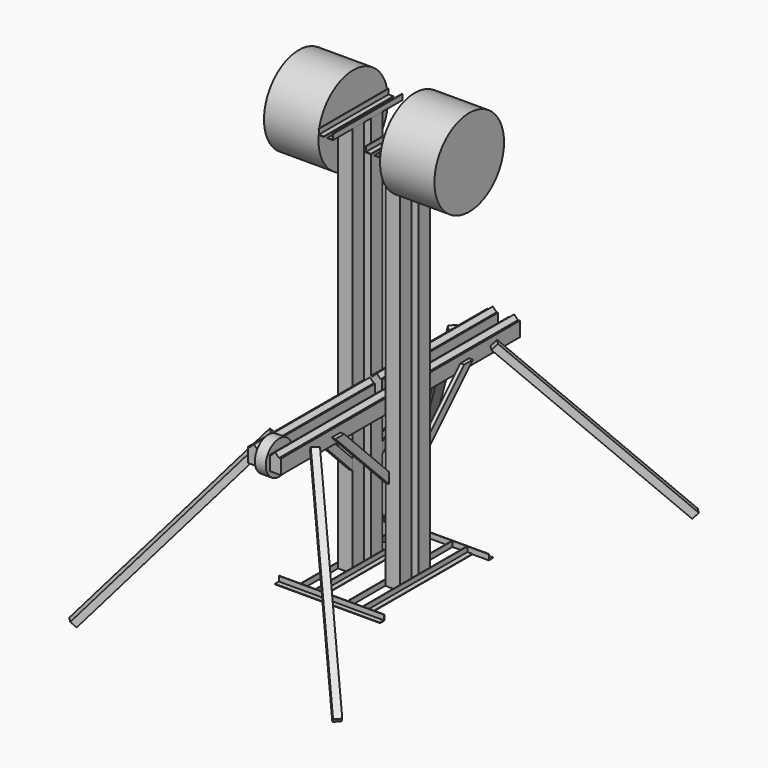
from build123d import *

# Parameters (mm, degrees)
F0_W      = 101.6
F0_H      = 101.6
F1_DEPTH  = 2743.2
F3_DEPTH  = 1016
F6_DEPTH  = 76.2
F8_DEPTH  = 26.924
F12_DEPTH = 457.2
F14_DEPTH = 368.3
F17_DEPTH = 304.8
F15_R     = 30.1625
F18_DEPTH = 381
F22_DEPTH = 50.8


with BuildPart() as f1:
    # F0 (on Top) → F1 (new body)
    with BuildSketch(Plane.XY):
        with Locations((-165.1, -80.9625)):
            Rectangle(F0_W, F0_H)
    extrude(amount=F1_DEPTH)


with BuildPart() as f1b:
    # F0 (on Top) → F1, piece 2 (new body)
    with BuildSketch(Plane.XY):
        with Locations((-165.1, 80.9625)):
            Rectangle(F0_W, F0_H)
    extrude(amount=F1_DEPTH)


with BuildPart() as f1c:
    # F0 (on Top) → F1, piece 3 (new body)
    with BuildSketch(Plane.XY):
        with Locations((165.1, 80.9625)):
            Rectangle(F0_W, F0_H)
    extrude(amount=F1_DEPTH)


with BuildPart() as f1d:
    # F0 (on Top) → F1, piece 4 (new body)
    with BuildSketch(Plane.XY):
        with Locations((165.1, -80.9625)):
            Rectangle(F0_W, F0_H)
    extrude(amount=F1_DEPTH)


with BuildPart() as f3:
    # F2 (on face) → F3 (new body)
    with BuildSketch(Plane.XZ.offset(-30.1625)):
        Polygon((-101.6, 1155.7), (-114.3, 1155.7), (-114.3, 1054.1), (-38.1, 1054.1), (-38.1, 1155.7), (-47.7184632736, 1155.7), align=None)
        Polygon((-74.6592316368, 1182.6407683632), (-101.6, 1155.7), (-47.7184632736, 1155.7), align=None)
    extrude(amount=-F3_DEPTH)


with BuildPart() as f3b:
    # F2 (on face) → F3, piece 2 (new body)
    with BuildSketch(Plane.XZ.offset(-30.1625)):
        Polygon((114.3, 1054.1), (114.3, 1155.7), (101.6, 1155.7), (47.7184632736, 1155.7), (38.1, 1155.7), (38.1, 1054.1), align=None)
        Polygon((47.7184632736, 1155.7), (101.6, 1155.7), (74.6592316368, 1182.6407683632), align=None)
    extrude(amount=-F3_DEPTH)


with BuildPart() as f4_1:
    # F4: instance of F3b
    add(f3b.part.mirror(Plane.XZ))


with BuildPart() as f4_2:
    # F4: instance of F3
    add(f3.part.mirror(Plane.XZ))


with BuildPart() as f6:
    # F5 (on face) → F6 (new body)
    with BuildSketch(Plane.YZ.offset(-38.1)):
        with BuildLine():
            ThreePointArc((-859.2767465332, 1054.1), (-850.6493347335, 1078.8515698747), (-847.725, 1104.9))
            ThreePointArc((-847.725, 1104.9), (-850.6493347335, 1130.9484301253), (-859.2767465332, 1155.7))
            Line((-859.2767465332, 1155.7), (-1046.1625, 1155.7))
            Line((-1046.1625, 1155.7), (-1046.1625, 1054.1))
            Line((-1046.1625, 1054.1), (-859.2767465332, 1054.1))
        make_face()
        with BuildLine():
            Line((-1046.1625, 1155.7), (-859.2767465332, 1155.7))
            ThreePointArc((-859.2767465332, 1155.7), (-1082.675, 1104.9), (-859.2767465332, 1054.1))
            Line((-859.2767465332, 1054.1), (-1046.1625, 1054.1))
            Line((-1046.1625, 1054.1), (-1046.1625, 1155.7))
        make_face()
    extrude(amount=F6_DEPTH)


with BuildPart() as f8:
    # F7 (on face) → F8 (new body)
    with BuildSketch(Plane.YZ.offset(114.3)):
        Polygon((-550.8625, 1054.1), (-131.7625, 635), (-131.7625, 711.1884929312), (-474.6740070688, 1054.1), align=None)
        Polygon((-601.6625, 1104.9), (-550.8625, 1054.1), (-474.6740070688, 1054.1), (-525.4740070688, 1104.9), align=None)
    extrude(amount=F8_DEPTH)


with BuildPart() as f9_1:
    # F9: instance of F8
    add(f8.part.mirror(Plane.XZ))


with BuildPart() as f10_1:
    # F10: instance of F8
    add(f8.part.mirror(Plane.YZ))


with BuildPart() as f10_2:
    # F10: instance of F9_1
    add(f9_1.part.mirror(Plane.YZ))


with BuildPart() as f12:
    # F11 (on Front) → F12 (new body, symmetric)
    with BuildSketch(Plane.XZ):
        Polygon((-254, 0), (-215.9, 0), (-215.9, 38.1), (-219.075, 38.1), (-219.075, 3.175), (-254, 3.175), align=None)
    extrude(amount=F12_DEPTH, both=True)


with BuildPart() as f12b:
    # F11 (on Front) → F12, piece 2 (new body, symmetric)
    with BuildSketch(Plane.XZ):
        Polygon((-114.3, 38.1), (-114.3, 0), (-76.2, 0), (-76.2, 3.175), (-111.125, 3.175), (-111.125, 38.1), align=None)
    extrude(amount=F12_DEPTH, both=True)


with BuildPart() as f12c:
    # F11 (on Front) → F12, piece 3 (new body, symmetric)
    with BuildSketch(Plane.XZ):
        Polygon((76.2, 0), (114.3, 0), (114.3, 38.1), (111.125, 38.1), (111.125, 3.175), (76.2, 3.175), align=None)
    extrude(amount=F12_DEPTH, both=True)


with BuildPart() as f12d:
    # F11 (on Front) → F12, piece 4 (new body, symmetric)
    with BuildSketch(Plane.XZ):
        Polygon((254, 0), (254, 3.175), (219.075, 3.175), (219.075, 38.1), (215.9, 38.1), (215.9, 0), align=None)
    extrude(amount=F12_DEPTH, both=True)


with BuildPart() as f14:
    # F13 (on Right) → F14 (new body, symmetric)
    with BuildSketch(Plane.YZ):
        Polygon((-495.3, 0), (-457.2, 0), (-457.2, 38.1), (-460.375, 38.1), (-460.375, 3.175), (-495.3, 3.175), align=None)
    extrude(amount=F14_DEPTH, both=True)


with BuildPart() as f14b:
    # F13 (on Right) → F14, piece 2 (new body, symmetric)
    with BuildSketch(Plane.YZ):
        Polygon((495.3, 0), (495.3, 3.175), (460.375, 3.175), (460.375, 38.1), (457.2, 38.1), (457.2, 0), align=None)
    extrude(amount=F14_DEPTH, both=True)


with BuildPart() as f17:
    # F16 (on Front) → F17 (new body, symmetric)
    with BuildSketch(Plane.XZ):
        Polygon((114.3, 2743.2), (152.4, 2743.2), (152.4, 2746.375), (117.475, 2746.375), (117.475, 2781.3), (114.3, 2781.3), align=None)
    extrude(amount=F17_DEPTH, both=True)


with BuildPart() as f17b:
    # F16 (on Front) → F17, piece 2 (new body, symmetric)
    with BuildSketch(Plane.XZ):
        Polygon((212.725, 2746.375), (177.8, 2746.375), (177.8, 2743.2), (215.9, 2743.2), (215.9, 2781.3), (212.725, 2781.3), align=None)
    extrude(amount=F17_DEPTH, both=True)


with BuildPart() as f17c:
    # F16 (on Front) → F17, piece 3 (new body, symmetric)
    with BuildSketch(Plane.XZ):
        Polygon((-215.9, 2781.3), (-215.9, 2743.2), (-177.8, 2743.2), (-177.8, 2746.375), (-212.725, 2746.375), (-212.725, 2781.3), align=None)
    extrude(amount=F17_DEPTH, both=True)


with BuildPart() as f17d:
    # F16 (on Front) → F17, piece 4 (new body, symmetric)
    with BuildSketch(Plane.XZ):
        Polygon((-152.4, 2743.2), (-114.3, 2743.2), (-114.3, 2781.3), (-117.475, 2781.3), (-117.475, 2746.375), (-152.4, 2746.375), align=None)
    extrude(amount=F17_DEPTH, both=True)


with BuildPart() as f18:
    # F15 (on face) → F18 (new body)
    with BuildSketch(Plane.YZ.offset(215.9)):
        with BuildLine():
            Line((30.1625, 2411.3210870781), (30.1625, 2714.625))
            Line((30.1625, 2714.625), (30.1625, 2743.2))
            Line((30.1625, 2743.2), (131.7625, 2743.2))
            Line((131.7625, 2743.2), (131.7625, 2439.7765261208))
            ThreePointArc((131.7625, 2439.7765261208), (257.9382193472, 2552.2337594727), (304.8, 2714.625))
            ThreePointArc((304.8, 2714.625), (-225.9386753081, 2919.2093469086), (30.1625, 2411.3210870781))
        make_face()
        with Locations((0, 2714.625)):
            Circle(F15_R, mode=Mode.SUBTRACT)
        with BuildLine():
            Line((30.1625, 2743.2), (30.1625, 2714.625))
            Line((30.1625, 2714.625), (30.1625, 2411.3210870781))
            ThreePointArc((30.1625, 2411.3210870781), (82.2031289491, 2421.1191472628), (131.7625, 2439.7765261208))
            Line((131.7625, 2439.7765261208), (131.7625, 2743.2))
            Line((131.7625, 2743.2), (30.1625, 2743.2))
        make_face()
        with Locations((0, 2714.625)):
            Circle(F15_R)
    extrude(amount=F18_DEPTH)


with BuildPart() as f19_1:
    # F19: instance of F18
    add(f18.part.mirror(Plane.YZ))


with BuildPart() as f22:
    # F21 (on face) → F22 (new body)
    with BuildSketch(Plane(origin=(338.1375, -338.1375, 0), x_dir=(-0.7071067812, -0.7071067812, 0), z_dir=(-0.7071067812, 0.7071067812, 0))):
        Polygon((675.199427547, 1140.8210244843), (639.2784030627, 1104.9), (1744.1784030627, 0), (1780.099427547, 35.9210244843), align=None)
    extrude(amount=F22_DEPTH)


with BuildPart() as f23_1:
    # F23: instance of F22
    add(f22.part.mirror(Plane.YZ))


with BuildPart() as f24_1:
    # F24: instance of F22
    add(f22.part.mirror(Plane.XZ))


with BuildPart() as f24_2:
    # F24: instance of F23_1
    add(f23_1.part.mirror(Plane.XZ))


solid = Compound([f1.part, f1b.part, f1c.part, f1d.part, f3.part, f3b.part, f4_1.part, f4_2.part, f6.part, f8.part, f9_1.part, f10_1.part, f10_2.part, f12.part, f12b.part, f12c.part, f12d.part, f14.part, f14b.part, f17.part, f17b.part, f17c.part, f17d.part, f18.part, f19_1.part, f22.part, f23_1.part, f24_1.part, f24_2.part])
